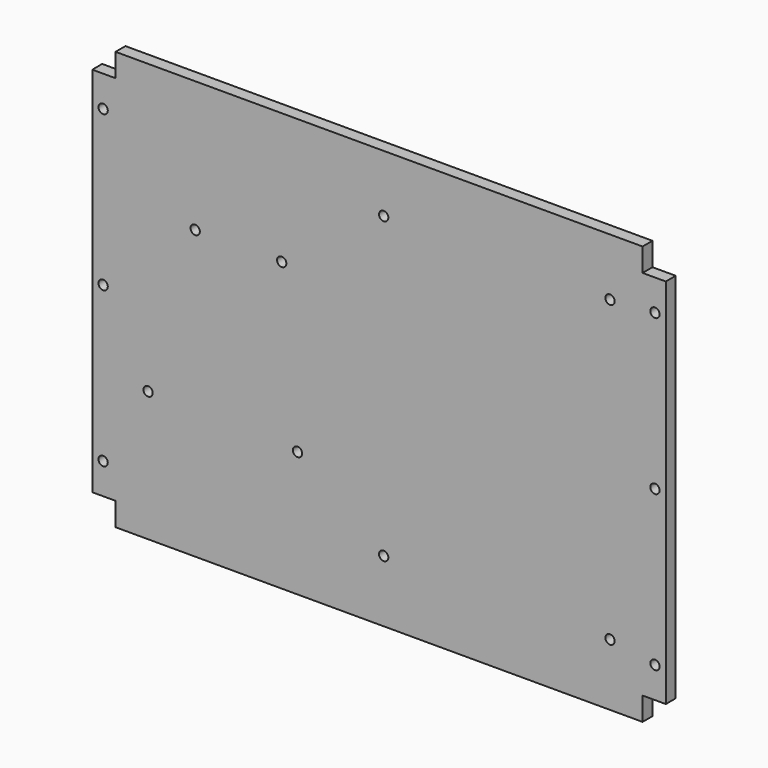
from build123d import *

# Parameters (mm, degrees)
F0_W     = 170
F0_H     = 7.5
F0_H_2   = 120
F0_W_2   = 7.5
F1_DEPTH = 4
F3_D     = 3
F5_D     = 3
F7_D     = 3


with BuildPart() as f1:
    # F0 (on Front) → F1 (new body)
    with BuildSketch(Plane.XZ):
        with Locations((92.5, 3.75)):
            Rectangle(F0_W, F0_H)
        with Locations((92.5, 67.5)):
            Rectangle(F0_W, F0_H_2)
        with Locations((3.75, 67.5)):
            Rectangle(F0_W_2, F0_H_2)
        with Locations((181.25, 67.5)):
            Rectangle(F0_W_2, F0_H_2)
        with Locations((92.5, 131.25)):
            Rectangle(F0_W, F0_H)
    extrude(amount=F1_DEPTH)

    # F3 (through all)
    with Locations(Plane.XZ.offset(4)):
        with Locations((3.5, 117.5), (3.5, 67.5), (3.5, 17.5), (181.5, 17.5), (181.5, 67.5), (181.5, 117.5)):
            Hole(F3_D / 2)

    # F5 (through all)
    with Locations(Plane.XZ.offset(4)):
        with Locations((94, 116.5), (167, 116.5), (167, 20), (94, 20)):
            Hole(F5_D / 2)

    # F7 (through all)
    with Locations(Plane.XZ.offset(4)):
        with Locations((18, 42), (33.2, 92.8), (61.1, 92.8), (66.2, 40.5)):
            Hole(F7_D / 2)


solid = f1.part
